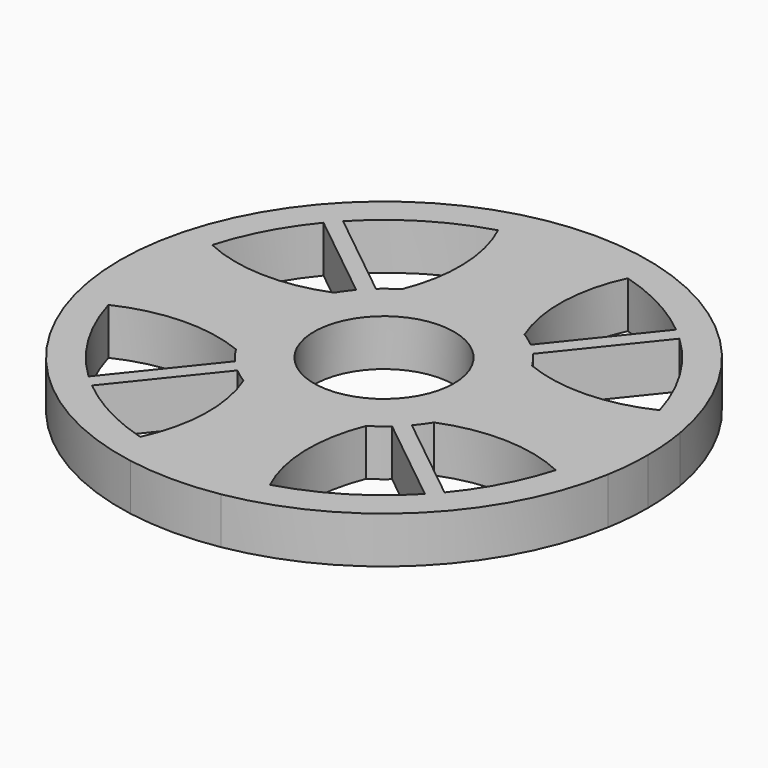
from build123d import *

# Parameters (mm, degrees)
F0_R     = 11.45
F1_DEPTH = 7.62


# Not quite as in the source:
# - a feature names something its author has since deleted; it is built from what else it names


with BuildPart() as f1:
    # F0 (on Top) → F1 (new body)
    with BuildSketch(Plane.XY):
        with BuildLine():
            ThreePointArc((-10.038027058, 16.1907539288), (0, 19.05), (10.038027058, 16.1907539288))
            ThreePointArc((10.038027058, 16.1907539288), (8.1892299167, 26.451450684), (10.618228457, 36.59047997))
            ThreePointArc((10.618228457, 36.59047997), (0, 38.1), (-10.618228457, 36.59047997))
            ThreePointArc((-10.618228457, 36.59047997), (-8.1892299167, 26.451450684), (-10.038027058, 16.1907539288))
        make_face()
        with BuildLine():
            ThreePointArc((16.1907539288, -10.038027058), (18.3212494435, -5.2186510544), (19.05, 0))
            ThreePointArc((19.05, 0), (18.3212494435, 5.2186510544), (16.1907539288, 10.038027058))
            ThreePointArc((16.1907539288, 10.038027058), (15.2571196867, 11.4071380664), (14.208032523, 12.6899295438))
            ThreePointArc((14.208032523, 12.6899295438), (13.3304286547, 13.6089004655), (12.3935124609, 14.4673200311))
            ThreePointArc((12.3935124609, 14.4673200311), (11.2488242673, 15.3742138857), (10.038027058, 16.1907539288))
            ThreePointArc((10.038027058, 16.1907539288), (0, 19.05), (-10.038027058, 16.1907539288))
            ThreePointArc((-10.038027058, 16.1907539288), (-11.4071380664, 15.2571196867), (-12.6899295437, 14.208032523))
            ThreePointArc((-12.6899295437, 14.208032523), (-13.6089004655, 13.3304286548), (-14.467320031, 12.3935124609))
            ThreePointArc((-14.467320031, 12.3935124609), (-15.3742138857, 11.2488242673), (-16.1907539288, 10.038027058))
            ThreePointArc((-16.1907539288, 10.038027058), (-19.05, 0), (-16.1907539288, -10.038027058))
            ThreePointArc((-16.1907539288, -10.038027058), (-15.2571196867, -11.4071380664), (-14.208032523, -12.6899295437))
            ThreePointArc((-14.208032523, -12.6899295437), (-13.3304286548, -13.6089004655), (-12.3935124609, -14.467320031))
            ThreePointArc((-12.3935124609, -14.467320031), (-11.2488242673, -15.3742138857), (-10.038027058, -16.1907539288))
            ThreePointArc((-10.038027058, -16.1907539288), (0, -19.05), (10.038027058, -16.1907539288))
            ThreePointArc((10.038027058, -16.1907539288), (11.4071380664, -15.2571196867), (12.6899295438, -14.208032523))
            ThreePointArc((12.6899295438, -14.208032523), (13.6089004655, -13.3304286547), (14.4673200311, -12.3935124609))
            ThreePointArc((14.4673200311, -12.3935124609), (15.3742138857, -11.2488242673), (16.1907539288, -10.038027058))
        make_face()
        Circle(F0_R, mode=Mode.SUBTRACT)
        with BuildLine():
            ThreePointArc((-10.618228457, 36.59047997), (0, 38.1), (10.618228457, 36.59047997))
            ThreePointArc((10.618228457, 36.59047997), (10.9631553547, 37.2915593412), (11.3294826074, 37.9816978733))
            ThreePointArc((11.3294826074, 37.9816978733), (9.6714472488, 40.5242467677), (7.4026469551, 42.5407242305))
            ThreePointArc((7.4026469551, 42.5407242305), (0, 43.18), (-7.4026469551, 42.5407242305))
            ThreePointArc((-7.4026469551, 42.5407242305), (-9.6714472488, 40.5242467677), (-11.3294826074, 37.9816978733))
            ThreePointArc((-11.3294826074, 37.9816978733), (-10.9631553547, 37.2915593412), (-10.618228457, 36.59047997))
        make_face()
        with BuildLine():
            ThreePointArc((-27.6564265836, 26.2055732359), (-19.8292429656, 32.5332310632), (-10.618228457, 36.59047997))
            ThreePointArc((-10.618228457, 36.59047997), (-10.9631553547, 37.2915593412), (-11.3294826074, 37.9816978733))
            ThreePointArc((-11.3294826074, 37.9816978733), (-9.6714472488, 40.5242467677), (-7.4026469551, 42.5407242305))
            ThreePointArc((-7.4026469551, 42.5407242305), (-30.5262465043, 30.5394936821), (-42.5375084691, 7.4211032363))
            ThreePointArc((-42.5375084691, 7.4211032363), (-42.4698240182, 7.5132687267), (-42.401220917, 7.6047524795))
            ThreePointArc((-42.401220917, 7.6047524795), (-40.430781391, 9.7510814924), (-37.9816978733, 11.3294826074))
            ThreePointArc((-37.9816978733, 11.3294826074), (-37.2915593412, 10.9631553547), (-36.59047997, 10.618228457))
            ThreePointArc((-36.59047997, 10.618228457), (-33.6685368778, 17.8336654815), (-29.3410352271, 24.3046014533))
            ThreePointArc((-29.3410352271, 24.3046014533), (-28.5145767397, 25.2691296517), (-27.6564265836, 26.2055732359))
        make_face()
        with BuildLine():
            ThreePointArc((-11.3294826074, -37.9816978733), (-10.9631553547, -37.2915593412), (-10.618228457, -36.59047997))
            ThreePointArc((-10.618228457, -36.59047997), (-17.8336654815, -33.6685368778), (-24.3046014533, -29.3410352271))
            ThreePointArc((-24.3046014533, -29.3410352271), (-25.2691296517, -28.5145767397), (-26.2055732359, -27.6564265836))
            ThreePointArc((-26.2055732359, -27.6564265836), (-32.5332310632, -19.8292429656), (-36.59047997, -10.618228457))
            ThreePointArc((-36.59047997, -10.618228457), (-37.2915593412, -10.9631553547), (-37.9816978733, -11.3294826074))
            ThreePointArc((-37.9816978733, -11.3294826074), (-40.5242467677, -9.6714472488), (-42.5407242305, -7.4026469551))
            ThreePointArc((-42.5407242305, -7.4026469551), (-30.5328708116, -30.5328708116), (-7.4026469551, -42.5407242305))
            ThreePointArc((-7.4026469551, -42.5407242305), (-9.6714472488, -40.5242467677), (-11.3294826074, -37.9816978733))
        make_face()
        with BuildLine():
            Line((-24.3046014533, -29.3410352271), (-12.3935124609, -14.467320031))
            ThreePointArc((-12.3935124609, -14.467320031), (-13.3304286548, -13.6089004655), (-14.208032523, -12.6899295437))
            Line((-14.208032523, -12.6899295437), (-26.2055732359, -27.6564265836))
            ThreePointArc((-26.2055732359, -27.6564265836), (-25.2691296517, -28.5145767397), (-24.3046014533, -29.3410352271))
        make_face()
        with BuildLine():
            ThreePointArc((10.6182284569, -36.59047997), (8.1892299167, -26.451450684), (10.038027058, -16.1907539288))
            ThreePointArc((10.038027058, -16.1907539288), (0, -19.05), (-10.038027058, -16.1907539288))
            ThreePointArc((-10.038027058, -16.1907539288), (-8.1892299167, -26.451450684), (-10.618228457, -36.59047997))
            ThreePointArc((-10.618228457, -36.59047997), (0, -38.1), (10.6182284569, -36.59047997))
        make_face()
        with BuildLine():
            ThreePointArc((11.3294826074, -37.9816978733), (10.9631553547, -37.2915593412), (10.6182284569, -36.59047997))
            ThreePointArc((10.6182284569, -36.59047997), (0, -38.1), (-10.618228457, -36.59047997))
            ThreePointArc((-10.618228457, -36.59047997), (-10.9631553547, -37.2915593412), (-11.3294826074, -37.9816978733))
            ThreePointArc((-11.3294826074, -37.9816978733), (-9.6714472488, -40.5242467677), (-7.4026469551, -42.5407242305))
            ThreePointArc((-7.4026469551, -42.5407242305), (0, -43.18), (7.4026469551, -42.5407242305))
            ThreePointArc((7.4026469551, -42.5407242305), (9.6714472488, -40.5242467677), (11.3294826074, -37.9816978733))
        make_face()
        with BuildLine():
            ThreePointArc((37.9816978733, 11.3294826074), (37.2915593412, 10.9631553547), (36.59047997, 10.6182284569))
            ThreePointArc((36.59047997, 10.6182284569), (37.7207322759, 5.3624953679), (38.1, 0))
            ThreePointArc((38.1, 0), (37.7207322759, -5.3624953679), (36.59047997, -10.618228457))
            ThreePointArc((36.59047997, -10.618228457), (37.2915593412, -10.9631553547), (37.9816978733, -11.3294826074))
            ThreePointArc((37.9816978733, -11.3294826074), (40.5242467677, -9.6714472488), (42.5407242305, -7.4026469551))
            ThreePointArc((42.5407242305, -7.4026469551), (43.0198841948, -3.7150994419), (43.18, 0))
            ThreePointArc((43.18, 0), (43.0198841948, 3.7150994419), (42.5407242305, 7.4026469551))
            ThreePointArc((42.5407242305, 7.4026469551), (40.5242467677, 9.6714472488), (37.9816978733, 11.3294826074))
        make_face()
        with BuildLine():
            ThreePointArc((16.1907539288, 10.038027058), (18.3212494435, 5.2186510544), (19.05, 0))
            ThreePointArc((19.05, 0), (18.3212494435, -5.2186510544), (16.1907539288, -10.038027058))
            ThreePointArc((16.1907539288, -10.038027058), (26.451450684, -8.1892299167), (36.59047997, -10.618228457))
            ThreePointArc((36.59047997, -10.618228457), (37.7207322759, -5.3624953679), (38.1, 0))
            ThreePointArc((38.1, 0), (37.7207322759, 5.3624953679), (36.59047997, 10.6182284569))
            ThreePointArc((36.59047997, 10.6182284569), (26.451450684, 8.1892299167), (16.1907539288, 10.038027058))
        make_face()
        with BuildLine():
            Line((29.3410352271, -24.3046014533), (14.467320031, -12.3935124609))
            ThreePointArc((14.4673200311, -12.3935124609), (13.6089004655, -13.3304286547), (12.6899295438, -14.208032523))
            Line((12.6899295437, -14.208032523), (27.6564265836, -26.2055732359))
            ThreePointArc((27.6564265836, -26.2055732359), (28.5145767397, -25.2691296517), (29.3410352271, -24.3046014533))
        make_face()
        with BuildLine():
            ThreePointArc((-14.467320031, 12.3935124609), (-13.6089004655, 13.3304286548), (-12.6899295437, 14.208032523))
            Line((-12.6899295437, 14.208032523), (-27.6564265836, 26.2055732359))
            ThreePointArc((-27.6564265836, 26.2055732359), (-28.5145767397, 25.2691296517), (-29.3410352271, 24.3046014533))
            Line((-29.3410352271, 24.3046014533), (-14.467320031, 12.3935124609))
        make_face()
        with BuildLine():
            ThreePointArc((12.3935124609, 14.4673200311), (13.3304286547, 13.6089004655), (14.208032523, 12.6899295438))
            Line((14.208032523, 12.6899295438), (26.2055732359, 27.6564265836))
            ThreePointArc((26.2055732359, 27.6564265836), (25.2691296517, 28.5145767397), (24.3046014533, 29.3410352271))
            Line((24.3046014533, 29.3410352271), (12.3935124609, 14.4673200311))
        make_face()
        with BuildLine():
            ThreePointArc((37.9816978733, -11.3294826074), (37.2915593412, -10.9631553547), (36.59047997, -10.618228457))
            ThreePointArc((36.59047997, -10.618228457), (33.6685368778, -17.8336654815), (29.3410352271, -24.3046014533))
            ThreePointArc((29.3410352271, -24.3046014533), (28.5145767397, -25.2691296517), (27.6564265836, -26.2055732359))
            ThreePointArc((27.6564265836, -26.2055732359), (19.8292429656, -32.5332310632), (10.6182284569, -36.59047997))
            ThreePointArc((10.6182284569, -36.59047997), (10.9631553547, -37.2915593412), (11.3294826074, -37.9816978733))
            ThreePointArc((11.3294826074, -37.9816978733), (9.6714472488, -40.5242467677), (7.4026469551, -42.5407242305))
            ThreePointArc((7.4026469551, -42.5407242305), (30.5328708116, -30.5328708116), (42.5407242305, -7.4026469551))
            ThreePointArc((42.5407242305, -7.4026469551), (40.5242467677, -9.6714472488), (37.9816978733, -11.3294826074))
        make_face()
        with BuildLine():
            ThreePointArc((26.2055732359, 27.6564265836), (32.5332310632, 19.8292429656), (36.59047997, 10.6182284569))
            ThreePointArc((36.59047997, 10.6182284569), (37.2915593412, 10.9631553547), (37.9816978733, 11.3294826074))
            ThreePointArc((37.9816978733, 11.3294826074), (40.5242467677, 9.6714472488), (42.5407242305, 7.4026469551))
            ThreePointArc((42.5407242305, 7.4026469551), (30.5328708116, 30.5328708116), (7.4026469551, 42.5407242305))
            ThreePointArc((7.4026469551, 42.5407242305), (9.6714472488, 40.5242467677), (11.3294826074, 37.9816978733))
            ThreePointArc((11.3294826074, 37.9816978733), (10.9631553547, 37.2915593412), (10.618228457, 36.59047997))
            ThreePointArc((10.618228457, 36.59047997), (17.8336654815, 33.6685368778), (24.3046014533, 29.3410352271))
            ThreePointArc((24.3046014533, 29.3410352271), (25.2691296517, 28.5145767397), (26.2055732359, 27.6564265836))
        make_face()
        with BuildLine():
            ThreePointArc((-16.1907539288, -10.038027058), (-19.05, 0), (-16.1907539288, 10.038027058))
            ThreePointArc((-16.1907539288, 10.038027058), (-26.451450684, 8.1892299167), (-36.59047997, 10.618228457))
            ThreePointArc((-36.59047997, 10.618228457), (-38.1, 0), (-36.59047997, -10.618228457))
            ThreePointArc((-36.59047997, -10.618228457), (-26.451450684, -8.1892299167), (-16.1907539288, -10.038027058))
        make_face()
        with BuildLine():
            ThreePointArc((-42.5407242305, 7.4026469551), (-43.18, 0), (-42.5407242305, -7.4026469551))
            ThreePointArc((-42.5407242305, -7.4026469551), (-40.5242467677, -9.6714472488), (-37.9816978733, -11.3294826074))
            ThreePointArc((-37.9816978733, -11.3294826074), (-37.2915593412, -10.9631553547), (-36.59047997, -10.618228457))
            ThreePointArc((-36.59047997, -10.618228457), (-38.1, 0), (-36.59047997, 10.618228457))
            ThreePointArc((-36.59047997, 10.618228457), (-37.2915593412, 10.9631553547), (-37.9816978733, 11.3294826074))
            ThreePointArc((-37.9816978733, 11.3294826074), (-40.430781391, 9.7510814924), (-42.401220917, 7.6047524795))
            ThreePointArc((-42.401220917, 7.6047524795), (-42.4715153756, 7.5040743862), (-42.5407242305, 7.4026469551))
        make_face()
    extrude(amount=F1_DEPTH)


solid = f1.part
